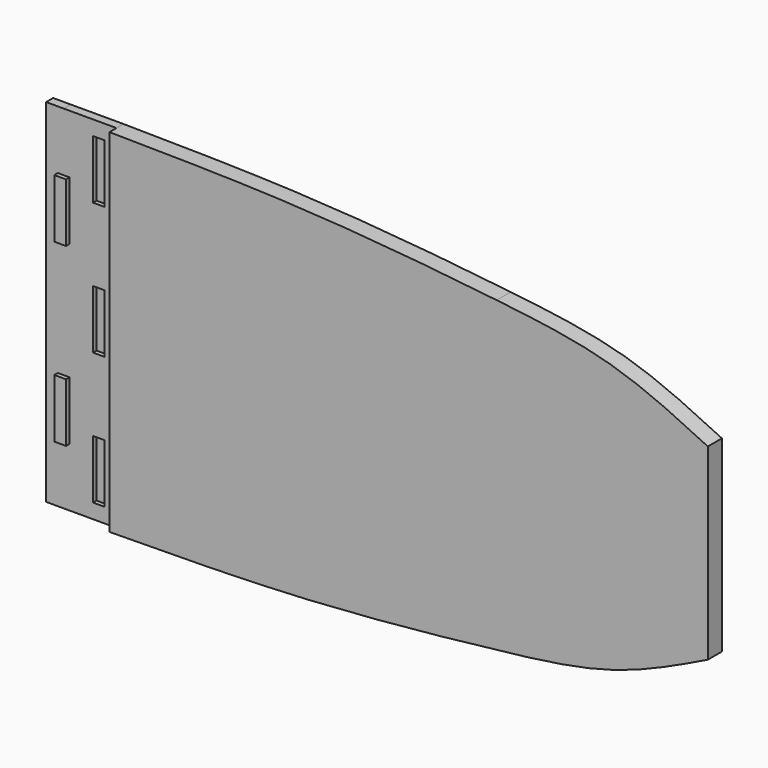
from build123d import *

# Parameters (mm, degrees)
F1_DEPTH = 19.05
F0_W     = 12.7
F0_H     = 63.5
F2_DEPTH = 9.525
F0_W_2   = 6.35
F0_H_2   = 31.75
F3_DEPTH = 4.7625
F4_DEPTH = 14.2875


# Not quite as in the source:
# - ends of sketch curves that miss each other by under 0.0002 mm in the source are joined


with BuildPart() as f1:
    # F0 (on Front) → F1 (new body)
    with BuildSketch(Plane.XZ):
        with BuildLine():
            Line((499.03344463, -13.7801575565), (499.03344463, -158.2426575565))
            add(Edge.make_bspline(
                [(499.03344463, -158.2426575565), (534.3674505865, -147.5744416568), (567.5004476082, -131.4772996066), (600.63344463, -115.3801575565)],
                knots=[0.7934300226, 0.7934300226, 0.7934300226, 0.7934300226, 1, 1, 1, 1], degree=3))
            Line((600.63344463, -115.3801575565), (600.63344463, -13.7801575565))
            Line((600.63344463, -13.7801575565), (600.63344463, 87.8198424435))
            add(Edge.make_bspline(
                [(600.63344463, 87.8198424435), (567.5002128258, 103.9114654586), (534.3669810216, 120.0030884738), (499.03344463, 130.6823424435)],
                knots=[0, 0, 0, 0, 0.2065722783, 0.2065722783, 0.2065722783, 0.2065722783], degree=3))
            Line((499.03344463, 130.6823424435), (499.03344463, -13.7801575565))
        make_face()
        with BuildLine():
            Line((169.2494543654, -13.9049269416), (169.2494543653, -198.8486769416))
            add(Edge.make_bspline(
                [(169.2494543653, -198.8486769416), (239.9344955626, -194.7900478461), (311.6955925282, -187.3813112289), (372.03344463, -180.4676575565)],
                knots=[0.2893668435, 0.2893668435, 0.2893668435, 0.2893668435, 0.5700660968, 0.5700660968, 0.5700660968, 0.5700660968], degree=3))
            Line((372.03344463, -180.4676575565), (372.03344463, -13.7801575565))
            Line((372.03344463, -13.7801575565), (372.03344463, 152.9073424435))
            add(Edge.make_bspline(
                [(372.03344463, 152.9073424435), (311.6965969023, 159.7662930053), (239.9327534215, 167.0025918958), (169.2494543654, 171.0388230584)],
                knots=[0.4299386922, 0.4299386922, 0.4299386922, 0.4299386922, 0.7106256488, 0.7106256488, 0.7106256488, 0.7106256488], degree=3))
            Line((169.2494543654, 171.0388230584), (169.2494543654, -13.9049269416))
        make_face()
        with BuildLine():
            Line((372.03344463, -13.7801575565), (372.03344463, -180.4676575565))
            add(Edge.make_bspline(
                [(372.03344463, -180.4676575565), (420.0467519851, -174.9661793441), (460.8268165983, -169.7781895634), (499.03344463, -158.2426575565)],
                knots=[0.5700660968, 0.5700660968, 0.5700660968, 0.5700660968, 0.7934300226, 0.7934300226, 0.7934300226, 0.7934300226], degree=3))
            Line((499.03344463, -158.2426575565), (499.03344463, -13.7801575565))
            Line((499.03344463, -13.7801575565), (499.03344463, 130.6823424435))
            add(Edge.make_bspline(
                [(499.03344463, 130.6823424435), (460.8273243383, 142.2298099053), (420.0485909934, 147.4490938355), (372.03344463, 152.9073424435)],
                knots=[0.2065722783, 0.2065722783, 0.2065722783, 0.2065722783, 0.4299386922, 0.4299386922, 0.4299386922, 0.4299386922], degree=3))
            Line((372.03344463, 152.9073424435), (372.03344463, -13.7801575565))
        make_face()
        with BuildLine():
            Line((-47.06655537, -13.7801514768), (-47.06655537, -204.2801485002))
            add(Edge.make_bspline(
                [(-47.06655537, -204.2801485002), (24.657602579, -203.6563895898), (96.3817605281, -203.0326306794), (169.2494543653, -198.8486769416)],
                knots=[0, 0, 0, 0, 0.2893668435, 0.2893668435, 0.2893668435, 0.2893668435], degree=3))
            Line((169.2494543653, -198.8486769416), (169.2494543654, -13.9049269416))
            Line((169.2494543654, -13.9049269416), (169.2494543654, 171.0388230584))
            add(Edge.make_bspline(
                [(169.2494543654, 171.0388230584), (96.3784736275, 175.1999774928), (24.6559591287, 175.9599115197), (-47.06655537, 176.7198455466)],
                knots=[0.7106256488, 0.7106256488, 0.7106256488, 0.7106256488, 1, 1, 1, 1], degree=3))
            Line((-47.06655537, 176.7198455466), (-47.06655537, -13.7801514768))
        make_face()
    extrude(amount=F1_DEPTH)

    # F0 (on Front) → F2 (join)
    with BuildSketch(Plane.XZ):
        Polygon((-123.26655537, 176.7198455466), (-123.26655537, -13.7801514768), (-104.21655537, -13.7801514768), (-104.21655537, 49.7198424435), (-110.56655537, 49.7198424435), (-110.56655537, 113.2198424435), (-104.21655537, 113.2198424435), (-104.21655537, 176.7198363638), align=None)
        Polygon((-104.21655537, 49.7198424435), (-104.21655537, -13.7801514768), (-85.16655537, -13.7801514768), (-85.16655537, 176.7198455466), (-104.21655537, 176.7198455466), (-104.21655537, 113.2198424435), (-97.86655537, 113.2198424435), (-97.86655537, 49.7198424435), align=None)
        Polygon((-85.16655537, 176.7198455466), (-85.16655537, -13.7801514768), (-72.46655537, -13.7801514768), (-72.46655537, 17.9698485232), (-66.11655537, 17.9698485232), (-66.11655537, 81.4698470349), (-66.11655537, 97.3448462908), (-72.46655537, 97.3448462908), (-72.46655537, 160.8448462908), (-66.11655537, 160.8448462908), (-66.11655537, 176.7198455466), align=None)
        Polygon((-47.06655537, 176.7198455466), (-66.11655537, 176.7198455466), (-66.11655537, 160.8448462908), (-59.76655537, 160.8448462908), (-59.76655537, 97.3448462908), (-66.11655537, 97.3448462908), (-66.11655537, 81.4698470349), (-66.11655537, 17.9698485232), (-59.76655537, 17.9698485232), (-59.76655537, -13.7801514768), (-47.06655537, -13.7801514768), align=None)
        Polygon((-104.21655537, -13.7801514768), (-123.26655537, -13.7801514768), (-123.26655537, -204.2801485003), (-104.21655537, -204.2801485002), (-104.21655537, -140.7801453971), (-110.56655537, -140.7801453971), (-110.56655537, -77.2801453971), (-104.21655537, -77.2801453971), align=None)
        Polygon((-85.16655537, -13.7801514768), (-104.21655537, -13.7801514768), (-104.21655537, -77.2801453971), (-97.86655537, -77.2801453971), (-97.86655537, -140.7801453971), (-104.21655537, -140.7801453971), (-104.21655537, -204.2801393175), (-85.16655537, -204.2801485002), align=None)
        Polygon((-72.46655537, -13.7801514768), (-85.16655537, -13.7801514768), (-85.16655537, -204.2801485002), (-47.06655537, -204.2801485002), (-47.06655537, -13.7801514768), (-59.76655537, -13.7801514768), (-59.76655537, -45.5301514768), (-66.11655537, -45.5301514768), (-72.46655537, -45.5301514768), align=None)
        with Locations((-66.11655537, -156.6551492444)):
            Rectangle(F0_W, F0_H, mode=Mode.SUBTRACT)
    extrude(amount=F2_DEPTH)

    # F0 (on Front) → F3 (join)
    with BuildSketch(Plane.XZ):
        with Locations((-66.11655537, -156.6551492444)):
            Rectangle(F0_W, F0_H)
        with Locations((-69.29155537, -29.6551514768)):
            Rectangle(F0_W_2, F0_H_2)
        with Locations((-62.94155537, -29.6551514768)):
            Rectangle(F0_W_2, F0_H_2)
        with Locations((-69.29155537, 2.0948485232)):
            Rectangle(F0_W_2, F0_H_2)
        with Locations((-62.94155537, 2.0948485232)):
            Rectangle(F0_W_2, F0_H_2)
        Polygon((-66.11655537, 129.0948462908), (-66.11655537, 160.8448462908), (-72.46655537, 160.8448462908), (-72.46655537, 97.3448462908), (-66.11655537, 97.3448462908), align=None)
        Polygon((-59.76655537, 160.8448462908), (-66.11655537, 160.8448462908), (-66.11655537, 129.0948462908), (-66.11655537, 97.3448462908), (-59.76655537, 97.3448462908), align=None)
    extrude(amount=F3_DEPTH)

    # F0 (on Front) → F4 (join)
    with BuildSketch(Plane.XZ):
        Polygon((-104.21655537, 81.4698424435), (-104.21655537, 49.7198424435), (-97.86655537, 49.7198424435), (-97.86655537, 113.2198424435), (-104.21655537, 113.2198424435), align=None)
        Polygon((-110.56655537, 49.7198424435), (-104.21655537, 49.7198424435), (-104.21655537, 81.4698424435), (-104.21655537, 113.2198424435), (-110.56655537, 113.2198424435), align=None)
        with Locations((-107.39155537, -109.0301453971)):
            Rectangle(F0_W_2, F0_H)
        with Locations((-101.04155537, -109.0301453971)):
            Rectangle(F0_W_2, F0_H)
    extrude(amount=F4_DEPTH)


solid = f1.part
